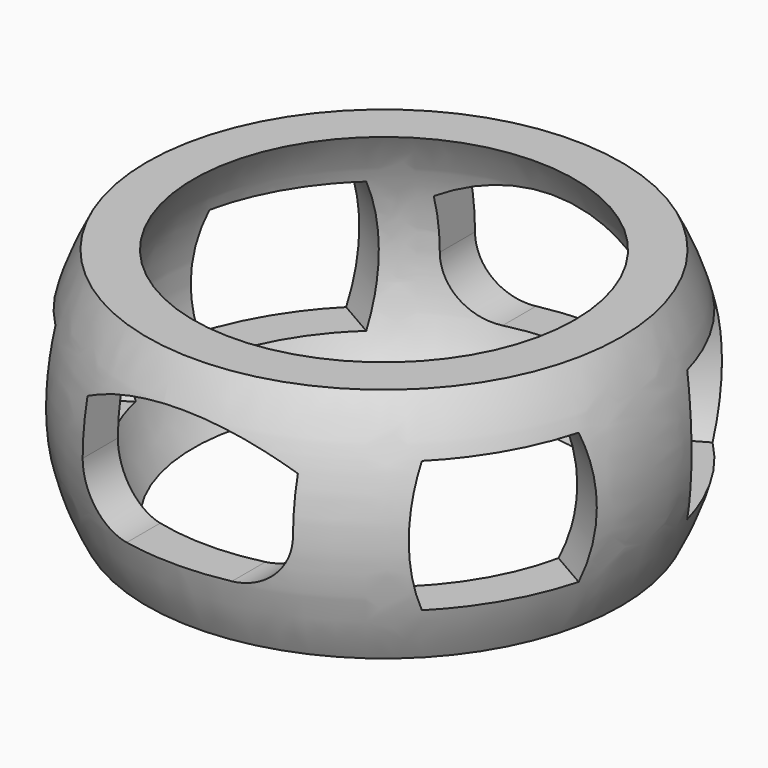
from build123d import *

# Parameters (mm, degrees)
F5_DEPTH  = 64.4460252684
F9_DEPTH  = 76.2402821611
F13_DEPTH = 94.8177659611


with BuildPart() as f2:
    # F1 (on Front) → F2 (revolve)
    with BuildSketch(Plane.XZ):
        with BuildLine():
            ThreePointArc((23.01875, 28.575), (27.4180989684, 14.2875), (23.01875, 0))
            Line((23.01875, 0), (28.6296326934, 0))
            ThreePointArc((28.6296326934, 0), (32.2225089684, 14.2875), (28.6296326934, 28.575))
            Line((28.6296326934, 28.575), (23.01875, 28.575))
        make_face()
    revolve(axis=Axis((0, 0, 14.2875), (0, 0, 1)))

    # F4 (on offset) → F5 (cut, through all)
    with BuildSketch(Plane.XZ.offset(32.2225162)):
        with BuildLine():
            Line((-6.35, 7.9375), (0, 7.9375))
            Line((0, 7.9375), (6.35, 7.9375))
            ThreePointArc((6.35, 7.9375), (10.8401280605, 9.7973719395), (12.7, 14.2875))
            Line((12.7, 14.2875), (12.7, 20.6375))
            Line((12.7, 20.6375), (-12.7, 20.6375))
            Line((-12.7, 20.6375), (-12.7, 14.2875))
            ThreePointArc((-12.7, 14.2875), (-10.8401280605, 9.7973719395), (-6.35, 7.9375))
        make_face()
        with BuildLine():
            Line((-12.7, 20.6375), (12.7, 20.6375))
            ThreePointArc((12.7, 20.6375), (0, 24.0404547439), (-12.7, 20.6375))
        make_face()
    extrude(amount=-F5_DEPTH, mode=Mode.SUBTRACT)

    # F8 (on face) → F9 (cut, through all)
    with BuildSketch(Plane(origin=(-27.9055176031, -16.1112581, 0), x_dir=(-0.5, 0.8660254038, 0), z_dir=(0.8660254038, 0.5, 0))):
        Polygon((-7.9375, 6.35), (0, 6.35), (0, 14.2875), (0, 22.225), (-7.9375, 22.225), align=None)
        Polygon((0, 14.2875), (0, 6.35), (7.9375, 6.35), (7.9375, 14.2875), (7.9375, 22.225), (0, 22.225), align=None)
        with BuildLine():
            Line((7.9375, 14.2875), (7.9375, 6.35))
            ThreePointArc((7.9375, 6.35), (9.5201471668, 14.2875), (7.9375, 22.225))
            Line((7.9375, 22.225), (7.9375, 14.2875))
        make_face()
        with BuildLine():
            ThreePointArc((-7.9375, 22.225), (-9.5201471668, 14.2875), (-7.9375, 6.35))
            Line((-7.9375, 6.35), (-7.9375, 22.225))
        make_face()
    extrude(amount=F9_DEPTH, mode=Mode.SUBTRACT)

    # F12 (on face) → F13 (cut, through all)
    with BuildSketch(Plane(origin=(-43.9940905122, 25.4, 0), x_dir=(-0.5, -0.8660254038, 0), z_dir=(-0.8660254038, 0.5, 0))):
        with BuildLine():
            Line((-7.9375, 6.35), (-7.9375, 14.2875))
            Line((-7.9375, 14.2875), (-7.9375, 22.225))
            ThreePointArc((-7.9375, 22.225), (-9.5201471668, 14.2875), (-7.9375, 6.35))
        make_face()
        Polygon((-7.9375, 22.225), (-7.9375, 14.2875), (-7.9375, 6.35), (0, 6.35), (0, 14.2875), (0, 22.225), align=None)
        Polygon((7.9375, 22.225), (0, 22.225), (0, 14.2875), (0, 6.35), (7.9375, 6.35), align=None)
        with BuildLine():
            ThreePointArc((7.9375, 6.35), (9.5201471668, 14.2875), (7.9375, 22.225))
            Line((7.9375, 22.225), (7.9375, 6.35))
        make_face()
    extrude(amount=-F13_DEPTH, mode=Mode.SUBTRACT)


solid = f2.part
